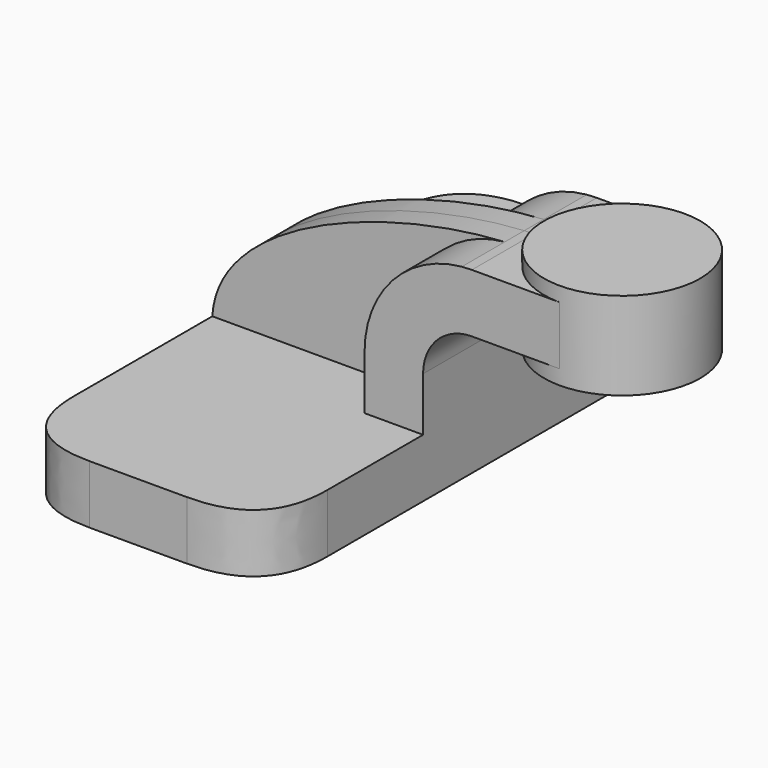
from build123d import *

# Parameters (mm, degrees)
F1_DEPTH    = 89.68002
F0_W        = 25.4
F0_H        = 19.05
F2_DEPTH    = 25.4
F3_DEPTH    = 7.9375
F5_T1_DEPTH = 146.05


# Not quite as in the source:
# - a fillet or chamfer that OpenCascade refuses, or shapes differently, is made with other operations: its cross-section is extruded or revolved along the edge and cut away or added


with BuildPart() as f1:
    # F0 (on Front) → F1 (new body, symmetric)
    with BuildSketch(Plane.XZ):
        Polygon((22.225, 9.525), (-41.275, 9.525), (-41.275, -9.525), (41.275, -9.525), (41.275, 9.525), align=None)
    extrude(amount=F1_DEPTH, both=True)

    # F0 (on Front) → F2 (join, symmetric)
    with BuildSketch(Plane.XZ):
        with BuildLine():
            Line((22.225, 27.0002), (22.225, 9.525))
            Line((22.225, 9.525), (41.275, 9.525))
            Line((41.275, 9.525), (41.275, 27.0002))
            ThreePointArc((41.275, 27.0002), (45.9246798487, 38.2255201513), (57.15, 42.8752))
            Line((57.15, 42.8752), (60.325, 42.8752))
            Line((60.325, 42.8752), (60.325, 61.9252))
            Line((60.325, 61.9252), (57.15, 61.9252))
            add(Edge.make_bspline(
                [(53.8854342407, 61.7722898912), (54.9842067368, 61.8365871986), (56.0728453275, 61.8876096574), (57.15, 61.9252)],
                knots=[108.5245810491, 108.5245810491, 108.5245810491, 108.5245810491, 111.5045361635, 111.5045361635, 111.5045361635, 111.5045361635], degree=3))
            ThreePointArc((53.8854342407, 61.7722898912), (31.3258777096, 50.5133948686), (22.225, 27.0002))
        make_face()
        with Locations((73.025, 52.4002)):
            Rectangle(F0_W, F0_H)
    extrude(amount=F2_DEPTH, both=True)

    # F0 (on Front) → F3 (join, symmetric)
    with BuildSketch(Plane.XZ):
        with BuildLine():
            add(Edge.make_bspline(
                [(-41.275, 9.525), (-39.5856284224, 39.4828766469), (13.870125209, 59.4306981306), (53.8854342407, 61.7722898912)],
                knots=[0, 0, 0, 0, 108.5245810491, 108.5245810491, 108.5245810491, 108.5245810491], degree=3))
            Line((-41.275, 9.525), (22.225, 9.525))
            Line((22.225, 9.525), (22.225, 27.0002))
            ThreePointArc((22.225, 27.0002), (31.3258777096, 50.5133948686), (53.8854342407, 61.7722898912))
        make_face()
    extrude(amount=F3_DEPTH, both=True)

    # F0 (on Front) → F4 (revolve)
    with BuildSketch(Plane.XZ):
        Polygon((85.725, 66.675), (85.725, 61.9252), (85.725, 42.8752), (85.725, 38.1), (111.125, 38.1), (111.125, 66.675), align=None)
    revolve(axis=Axis((85.725, 0, 52.3875), (0, 0, 1)))

    # F5: fillet of radius 25.4 on 4 edges, made by hand

    # F5_s2 → F5_t1 (cut)
    with BuildSketch(Plane.XY.offset(-73.025)):
        with BuildLine():
            add(Edge.make_bspline(
                [(41.275, -64.28002), (41.275, -89.68002), (15.875, -89.68002)],
                knots=[0, 0, 0, 1, 1, 1], degree=2, weights=[1, 1, 1]))
            Line((15.875, -89.68002), (41.275, -89.68002))
            Line((41.275, -89.68002), (41.275, -64.28002))
        make_face()
        with BuildLine():
            add(Edge.make_bspline(
                [(-41.275, -64.28002), (-41.275, -89.68002), (-15.875, -89.68002)],
                knots=[0, 0, 0, 1, 1, 1], degree=2, weights=[1, 1, 1]))
            Line((-15.875, -89.68002), (-41.275, -89.68002))
            Line((-41.275, -89.68002), (-41.275, -64.28002))
        make_face()
        with BuildLine():
            add(Edge.make_bspline(
                [(41.275, 64.28002), (41.275, 89.68002), (15.875, 89.68002)],
                knots=[0, 0, 0, 1, 1, 1], degree=2, weights=[1, 1, 1]))
            Line((15.875, 89.68002), (41.275, 89.68002))
            Line((41.275, 89.68002), (41.275, 64.28002))
        make_face()
        with BuildLine():
            add(Edge.make_bspline(
                [(-41.275, 64.28002), (-41.275, 89.68002), (-15.875, 89.68002)],
                knots=[0, 0, 0, 1, 1, 1], degree=2, weights=[1, 1, 1]))
            Line((-15.875, 89.68002), (-41.275, 89.68002))
            Line((-41.275, 89.68002), (-41.275, 64.28002))
        make_face()
    extrude(amount=F5_T1_DEPTH, mode=Mode.SUBTRACT)


solid = f1.part
